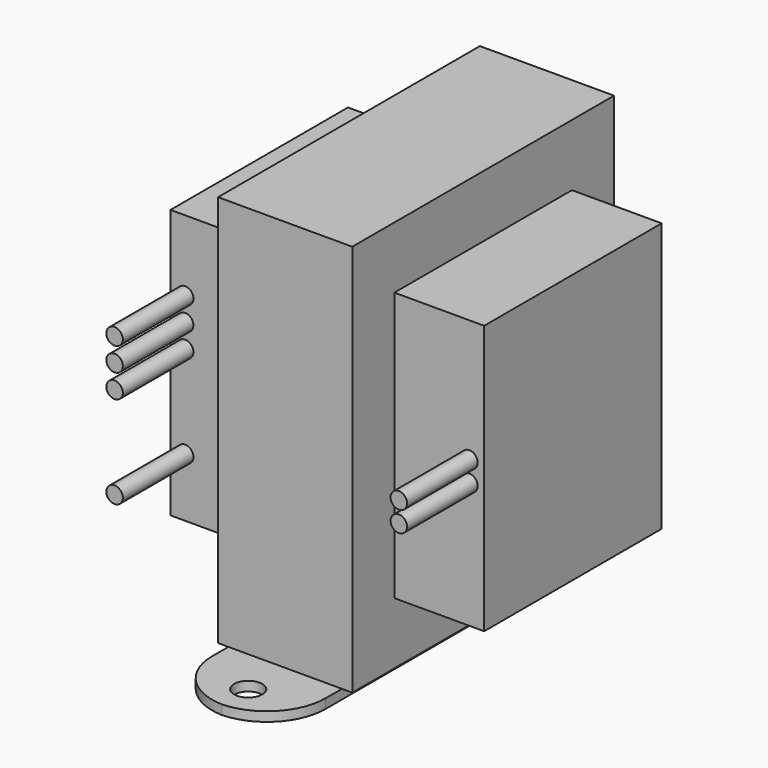
from build123d import *

# Parameters (mm, degrees)
F0_W         = 19.3
F0_H         = 82.5
F1_DEPTH     = 1.6
F2_W         = 22.8
F2_H         = 55.6
F3_DEPTH     = 66.7
F4_W         = 37.7
F4_H         = 45.7
F5_DEPTH     = 15.25
F6_W         = 37.7
F6_H         = 45.7
F7_DEPTH     = 15.25
F8_R         = 2.4
F9_DEPTH     = 68.301
F10_T1_DEPTH = 51.6
F11_R        = 1.4
F12_DEPTH    = 15
F13_R        = 1.4
F14_DEPTH    = 15


# Not quite as in the source:
# - a fillet or chamfer that OpenCascade refuses, or shapes differently, is made with other operations: its cross-section is extruded or revolved along the edge and cut away or added


with BuildPart() as f1:
    # F0 (on Top) → F1 (new body)
    with BuildSketch(Plane.XY):
        Rectangle(F0_W, F0_H)
    extrude(amount=F1_DEPTH)

    # F2 (on face) → F3 (join)
    with BuildSketch(Plane.XY.offset(1.6)):
        Rectangle(F2_W, F2_H)
    extrude(amount=F3_DEPTH)

    # F4 (on face) → F5 (join)
    with BuildSketch(Plane(origin=(-11.4, 0, 0), x_dir=(0, -1, 0), z_dir=(-1, 0, 0))):
        with Locations((0, 34.95)):
            Rectangle(F4_W, F4_H)
    extrude(amount=F5_DEPTH)

    # F6 (on face) → F7 (join)
    with BuildSketch(Plane.YZ.offset(11.4)):
        with Locations((0, 34.95)):
            Rectangle(F6_W, F6_H)
    extrude(amount=F7_DEPTH)

    # F8 (on face) → F9 (cut, through all)
    with BuildSketch(Plane(origin=(0, 0, 0), x_dir=(1, 0, 0), z_dir=(0, 0, -1))):
        with Locations((0, 35.65)):
            Circle(F8_R)
        with Locations((0, -35.65)):
            Circle(F8_R)
    extrude(amount=-F9_DEPTH, mode=Mode.SUBTRACT)

    # F10: fillet of radius 10 on 4 edges, made by hand

    # F10_s2 → F10_t1 (cut)
    with BuildSketch(Plane.XY.offset(-25)):
        with BuildLine():
            ThreePointArc((0.35, 41.25), (-6.7210678119, 38.3210678119), (-9.65, 31.25))
            Line((-9.65, 31.25), (-9.65, 41.25))
            Line((-9.65, 41.25), (0.35, 41.25))
        make_face()
        with BuildLine():
            ThreePointArc((9.65, 31.25), (6.7210678119, 38.3210678119), (-0.35, 41.25))
            Line((-0.35, 41.25), (9.65, 41.25))
            Line((9.65, 41.25), (9.65, 31.25))
        make_face()
        with BuildLine():
            ThreePointArc((9.65, -31.25), (6.7210678119, -38.3210678119), (-0.35, -41.25))
            Line((-0.35, -41.25), (9.65, -41.25))
            Line((9.65, -41.25), (9.65, -31.25))
        make_face()
        with BuildLine():
            ThreePointArc((0.35, -41.25), (-6.7210678119, -38.3210678119), (-9.65, -31.25))
            Line((-9.65, -31.25), (-9.65, -41.25))
            Line((-9.65, -41.25), (0.35, -41.25))
        make_face()
    extrude(amount=F10_T1_DEPTH, mode=Mode.SUBTRACT)

    # F11 (on face) → F12 (join)
    with BuildSketch(Plane.XZ.offset(18.85)):
        with Locations((-24.15, 41.8)):
            Circle(F11_R)
        with Locations((-24.15, 45.8)):
            Circle(F11_R)
        with Locations((-24.15, 37.8)):
            Circle(F11_R)
        with Locations((-24.15, 22.1)):
            Circle(F11_R)
    extrude(amount=F12_DEPTH)

    # F13 (on face) → F14 (join)
    with BuildSketch(Plane.XZ.offset(18.85)):
        with Locations((24.15, 36.9742031991)):
            Circle(F13_R)
        with Locations((24.15, 33.4742031991)):
            Circle(F13_R)
    extrude(amount=F14_DEPTH)


solid = f1.part
